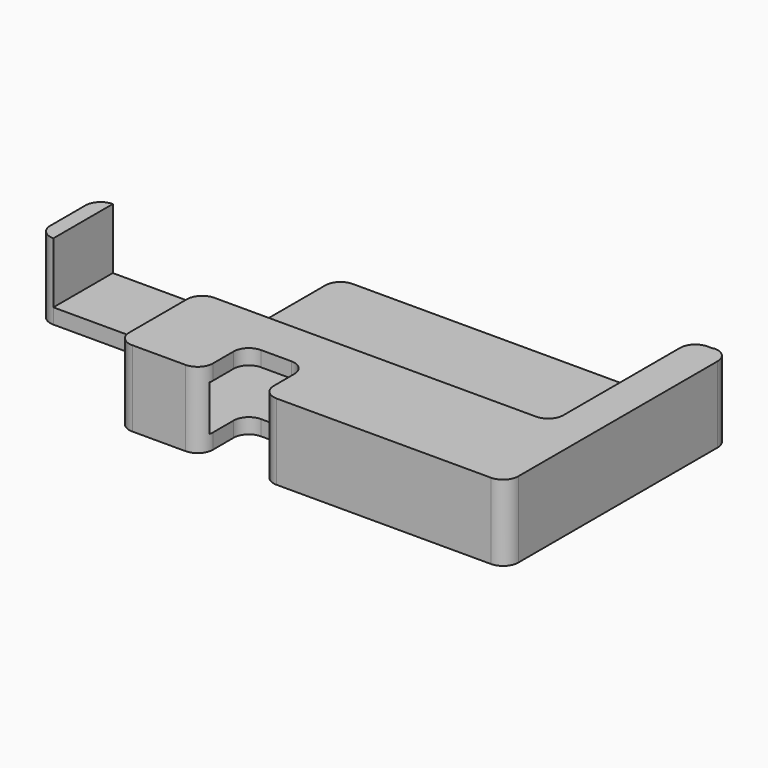
from build123d import *

# Parameters (mm, degrees)
F1_DEPTH     = 25
F4_DEPTH     = 25
F6_DEPTH     = 20
F7_W         = 51.9104144033
F7_H         = 33.7755738664
F7_W_2       = 52.9833799657
F8_DEPTH     = 25
F9_W         = 5
F9_H         = 24.4488522671
F10_DEPTH    = 20
F11_W        = 120.8302378654
F11_H        = 15
F12_DEPTH    = 30
F14_DEPTH    = 6
F15_R        = 7.2754238601
F15_R_2      = 3.5
F15_R_3      = 6.751082942
F16_DEPTH    = 2
F17_W        = 5
F17_H        = 5
F18_DEPTH    = 58
F19_DEPTH    = 2
F20_T1_DEPTH = 5
F20_T3_DEPTH = 5
F20_T5_DEPTH = 50
F20_T7_DEPTH = 30
F20_T9_DEPTH = 30


# Not quite as in the source:
# - a fillet or chamfer that OpenCascade refuses, or shapes differently, is made with other operations: its cross-section is extruded or revolved along the edge and cut away or added
# - a feature names something its author has since deleted; it is built from what else it names


with BuildPart() as f1:
    # F0 (on Top) → F1 (new body)
    with BuildSketch(Plane.XY):
        Polygon((-25, 55.486739397), (-90.4999962505, 55.486739397), (-90.4999962505, -36.513260603), (90.5000037495, -36.513260603), (90.5000037495, 55.486739397), (25, 55.486739397), align=None)
    extrude(amount=F1_DEPTH)

    # F3 (on face) → F4 (cut)
    with BuildSketch(Plane.XY.offset(25)):
        Polygon((10, -17.952421695), (0, -17.952421695), (-10, -17.952421695), (-10, -30.3189372783), (0, -30.3189372783), (10, -30.3189372783), align=None)
        Polygon((10, -36.513260603), (10, -30.3189372783), (0, -30.3189372783), (-10, -30.3189372783), (-10, -36.513260603), align=None)
    extrude(amount=-F4_DEPTH, mode=Mode.SUBTRACT)

    # F5 (on face) → F6 (cut)
    with BuildSketch(Plane.XY.offset(25)):
        Polygon((83.3136215806, -2.7376867365), (83.3136215806, 55.486739397), (-90.4999962505, 55.486739397), (-90.4999962505, -36.513260603), (-37.5166162848, -36.513260603), (-37.5166162848, -2.7376867365), align=None)
    extrude(amount=-F6_DEPTH, mode=Mode.SUBTRACT)

    # F7 (on face) → F8 (cut)
    with BuildSketch(Plane.XY.offset(5)):
        with Locations((-64.5447890489, 38.5989524638)):
            Rectangle(F7_W, F7_H)
        with Locations((-64.0083062677, -19.6254736697)):
            Rectangle(F7_W_2, F7_H)
    extrude(amount=-F8_DEPTH, mode=Mode.SUBTRACT)

    # F9 (on face) → F10 (join)
    with BuildSketch(Plane.XY.offset(5)):
        with Locations((-87.9999962505, 9.486739397)):
            Rectangle(F9_W, F9_H)
    extrude(amount=F10_DEPTH)

    # F11 (on face) → F12 (cut)
    with BuildSketch(Plane(origin=(0, -2.7376867365, 0), x_dir=(-1, 0, 0), z_dir=(0, 1, 0))):
        with Locations((-22.8985026479, 12.5)):
            Rectangle(F11_W, F11_H)
    extrude(amount=-F12_DEPTH, mode=Mode.SUBTRACT)

    # F13 (on face) → F14 (cut)
    with BuildSketch(Plane.XY.offset(5)):
        with BuildLine():
            ThreePointArc((64.3544293493, 12.8630390391), (60.8544293493, 16.3630390391), (57.3544293493, 12.8630390391))
            Line((57.3544293493, 12.8630390391), (60.8544293493, 12.8630390391))
            Line((60.8544293493, 12.8630390391), (64.3544293493, 12.8630390391))
        make_face()
        with BuildLine():
            Line((60.8544293493, 12.8630390391), (57.3544293493, 12.8630390391))
            ThreePointArc((57.3544293493, 12.8630390391), (60.8544293493, 9.3630390391), (64.3544293493, 12.8630390391))
            Line((64.3544293493, 12.8630390391), (60.8544293493, 12.8630390391))
        make_face()
        with BuildLine():
            ThreePointArc((-23.8955706507, 12.8630390391), (-27.3955706507, 16.3630390391), (-30.8955706507, 12.8630390391))
            Line((-30.8955706507, 12.8630390391), (-27.3955706507, 12.8630390391))
            Line((-27.3955706507, 12.8630390391), (-23.8955706507, 12.8630390391))
        make_face()
        with BuildLine():
            Line((-27.3955706507, 12.8630390391), (-30.8955706507, 12.8630390391))
            ThreePointArc((-30.8955706507, 12.8630390391), (-27.3955706507, 9.3630390391), (-23.8955706507, 12.8630390391))
            Line((-23.8955706507, 12.8630390391), (-27.3955706507, 12.8630390391))
        make_face()
    extrude(amount=-F14_DEPTH, mode=Mode.SUBTRACT)

    # F15 (on face) → F16 (cut)
    with BuildSketch(Plane.XY.offset(5)):
        with Locations((60.8544293493, 12.8630390391)):
            Circle(F15_R)
        with Locations((60.8544293493, 12.8630390391)):
            Circle(F15_R_2, mode=Mode.SUBTRACT)
        with Locations((-27.3955706507, 12.8630390391)):
            Circle(F15_R_3)
        with Locations((-27.3955706507, 12.8630390391)):
            Circle(F15_R_2, mode=Mode.SUBTRACT)
    extrude(amount=-F16_DEPTH, mode=Mode.SUBTRACT)

    # F17 (on face) → F18 (join)
    with BuildSketch(Plane(origin=(0, -2.7376867365, 0), x_dir=(-1, 0, 0), z_dir=(0, 1, 0))):
        with Locations((-80.8136215806, 22.5)):
            Rectangle(F17_W, F17_H)
    extrude(amount=F18_DEPTH)

    # F19 (cut): a face of the model
    f19_faces = [f1.faces().sort_by_distance(p)[0] for p in [
        (83.3136215806, 11.4118039273, 12.5084721811),
    ]]
    extrude(f19_faces, amount=-F19_DEPTH, mode=Mode.SUBTRACT)

    # F20: fillet of radius 5 on 17 edges, made by hand

    # F20_s2 → F20_t1 (join)
    with BuildSketch(Plane.XY.offset(20)):
        with BuildLine():
            ThreePointArc((-10, -22.952421695), (-8.5355339059, -19.4168877891), (-5, -17.952421695))
            Line((-5, -17.952421695), (-10, -17.952421695))
            Line((-10, -17.952421695), (-10, -22.952421695))
        make_face()
        with BuildLine():
            ThreePointArc((5, -17.952421695), (8.5355339059, -19.4168877891), (10, -22.952421695))
            Line((10, -22.952421695), (10, -17.952421695))
            Line((10, -17.952421695), (5, -17.952421695))
        make_face()
        with BuildLine():
            ThreePointArc((78.3136215806, 2.2623132635), (76.8491554865, -1.2732206424), (73.3136215806, -2.7376867365))
            Line((73.3136215806, -2.7376867365), (78.3136215806, -2.7376867365))
            Line((78.3136215806, -2.7376867365), (78.3136215806, 2.2623132635))
        make_face()
    extrude(amount=F20_T1_DEPTH)

    # F20_s4 → F20_t3 (join)
    with BuildSketch(Plane.XY):
        with BuildLine():
            ThreePointArc((-10, -22.952421695), (-8.5355339059, -19.4168877891), (-5, -17.952421695))
            Line((-5, -17.952421695), (-10, -17.952421695))
            Line((-10, -17.952421695), (-10, -22.952421695))
        make_face()
        with BuildLine():
            ThreePointArc((10, -22.952421695), (8.5355339059, -19.4168877891), (5, -17.952421695))
            Line((5, -17.952421695), (10, -17.952421695))
            Line((10, -17.952421695), (10, -22.952421695))
        make_face()
        with BuildLine():
            ThreePointArc((-42.5166162848, -2.7376867365), (-38.9810823789, -4.2021528306), (-37.5166162848, -7.7376867365))
            Line((-37.5166162848, -7.7376867365), (-37.5166162848, -2.7376867365))
            Line((-37.5166162848, -2.7376867365), (-42.5166162848, -2.7376867365))
        make_face()
        with BuildLine():
            ThreePointArc((-38.5895818472, 26.7111655306), (-40.0540479413, 23.1756316247), (-43.5895818472, 21.7111655306))
            Line((-43.5895818472, 21.7111655306), (-38.5895818472, 21.7111655306))
            Line((-38.5895818472, 21.7111655306), (-38.5895818472, 26.7111655306))
        make_face()
    extrude(amount=F20_T3_DEPTH)

    # F20_s6 → F20_t5 (cut)
    with BuildSketch(Plane.XY.offset(-12.5)):
        with BuildLine():
            ThreePointArc((-10, -31.513260603), (-11.4644660941, -35.0487945089), (-15, -36.513260603))
            Line((-15, -36.513260603), (-10, -36.513260603))
            Line((-10, -36.513260603), (-10, -31.513260603))
        make_face()
        with BuildLine():
            ThreePointArc((15, -36.513260603), (11.4644660941, -35.0487945089), (10, -31.513260603))
            Line((10, -31.513260603), (10, -36.513260603))
            Line((10, -36.513260603), (15, -36.513260603))
        make_face()
        with BuildLine():
            ThreePointArc((-32.5166162848, -36.513260603), (-36.0521501908, -35.0487945089), (-37.5166162848, -31.513260603))
            Line((-37.5166162848, -31.513260603), (-37.5166162848, -36.513260603))
            Line((-37.5166162848, -36.513260603), (-32.5166162848, -36.513260603))
        make_face()
        with BuildLine():
            ThreePointArc((90.5000037495, 50.486739397), (89.0355376554, 54.022273303), (85.5000037495, 55.486739397))
            Line((85.5000037495, 55.486739397), (90.5000037495, 55.486739397))
            Line((90.5000037495, 55.486739397), (90.5000037495, 50.486739397))
        make_face()
        with BuildLine():
            ThreePointArc((90.5000037495, -31.513260603), (89.0355376554, -35.0487945089), (85.5000037495, -36.513260603))
            Line((85.5000037495, -36.513260603), (90.5000037495, -36.513260603))
            Line((90.5000037495, -36.513260603), (90.5000037495, -31.513260603))
        make_face()
        with BuildLine():
            ThreePointArc((-90.4999962505, 16.7111655306), (-89.0355301565, 20.2466994365), (-85.4999962505, 21.7111655306))
            Line((-85.4999962505, 21.7111655306), (-90.4999962505, 21.7111655306))
            Line((-90.4999962505, 21.7111655306), (-90.4999962505, 16.7111655306))
        make_face()
        with BuildLine():
            ThreePointArc((-90.4999962505, 2.2623132635), (-89.0355301565, -1.2732206424), (-85.4999962505, -2.7376867365))
            Line((-85.4999962505, -2.7376867365), (-90.4999962505, -2.7376867365))
            Line((-90.4999962505, -2.7376867365), (-90.4999962505, 2.2623132635))
        make_face()
    extrude(amount=F20_T5_DEPTH, mode=Mode.SUBTRACT)

    # F20_s8 → F20_t7 (cut)
    with BuildSketch(Plane.XY.offset(-12.5)):
        with BuildLine():
            ThreePointArc((-33.5895818472, 55.486739397), (-37.1251157531, 54.022273303), (-38.5895818472, 50.486739397))
            Line((-38.5895818472, 50.486739397), (-38.5895818472, 55.486739397))
            Line((-38.5895818472, 55.486739397), (-33.5895818472, 55.486739397))
        make_face()
    extrude(amount=F20_T7_DEPTH, mode=Mode.SUBTRACT)

    # F20_s10 → F20_t9 (cut)
    with BuildSketch(Plane.XY.offset(7.5)):
        with BuildLine():
            ThreePointArc((83.3136215806, 55.2623132635), (79.7780876747, 53.7978471694), (78.3136215806, 50.2623132635))
            Line((78.3136215806, 50.2623132635), (78.3136215806, 55.2623132635))
            Line((78.3136215806, 55.2623132635), (83.3136215806, 55.2623132635))
        make_face()
        with BuildLine():
            ThreePointArc((-37.5166162848, -7.7376867365), (-36.0521501908, -4.2021528306), (-32.5166162848, -2.7376867365))
            Line((-32.5166162848, -2.7376867365), (-37.5166162848, -2.7376867365))
            Line((-37.5166162848, -2.7376867365), (-37.5166162848, -7.7376867365))
        make_face()
    extrude(amount=F20_T9_DEPTH, mode=Mode.SUBTRACT)


solid = f1.part
